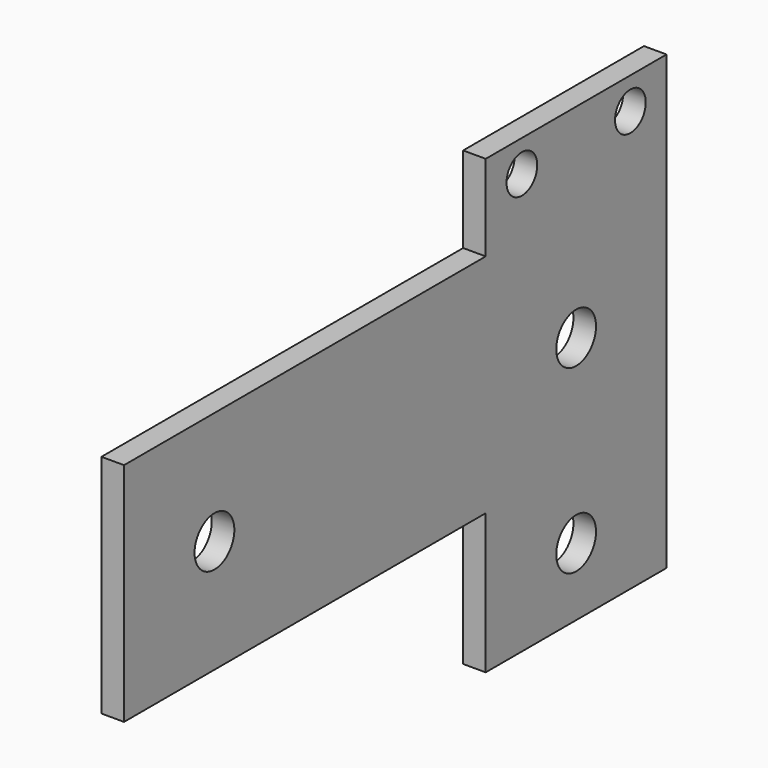
from build123d import *

# Parameters (mm, degrees)
F1_DEPTH = 5
F2_D     = 8.5
F3_D     = 11


# Not quite as in the source:
# - a feature names something its author has since deleted; it is built from what else it names


with BuildPart() as f1:
    # F0 (on Right) → F1 (new body)
    with BuildSketch(Plane.YZ):
        Polygon((31.0329496861, 74.6778247207), (-18.9670503139, 74.6778247207), (-18.9670503139, 55.6778247207), (-118.9670503139, 55.6778247207), (-118.9670503139, 5.6778247207), (-18.9670503139, 5.6778247207), (-18.9670503139, -25.3221752793), (31.0329496861, -25.3221752793), align=None)
    extrude(amount=F1_DEPTH)

    # F2 (through all)
    with Locations(Plane(origin=(0, 0, 0), x_dir=(0, 1, 0), z_dir=(-1, 0, 0))):
        with Locations((-8.9670503139, -67.6778247207), (21.0329496861, -67.6778247207)):
            Hole(F2_D / 2)

    # F3 (through all)
    with Locations(Plane(origin=(0, 0, 0), x_dir=(0, 1, 0), z_dir=(-1, 0, 0))):
        with Locations((6.0329496861, -29.6778247207), (6.0329496861, 10.3221752793), (-93.9670503139, -30.6778247207)):
            Hole(F3_D / 2)


solid = f1.part
